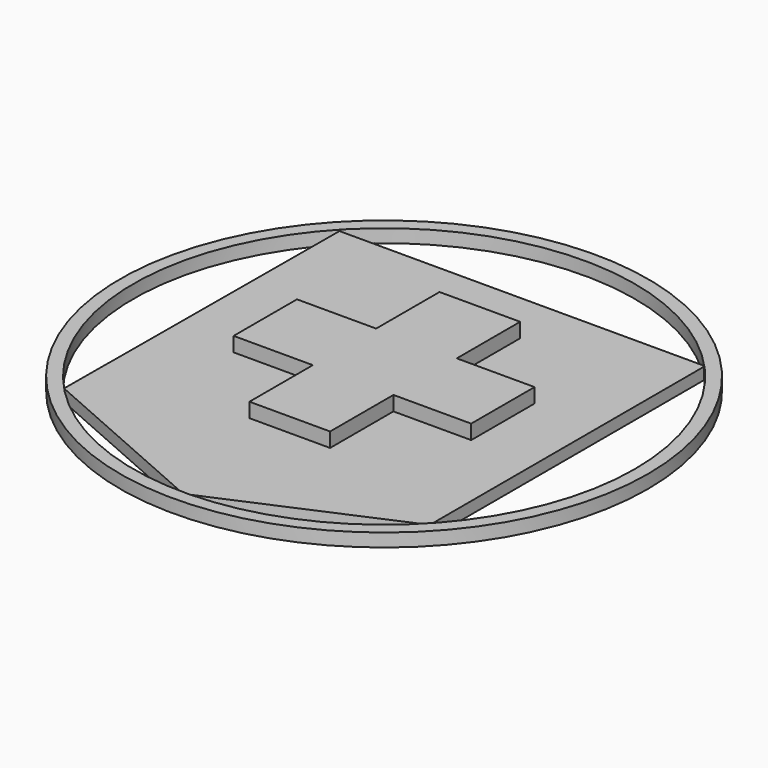
from build123d import *

# Parameters (mm, degrees)
F0_R     = 20
F0_R_2   = 19
F1_DEPTH = 1
F3_W     = 3
F3_H     = 3
F3_H_2   = 2.9973080382
F4_DEPTH = 2
F5_DEPTH = 0.9


with BuildPart() as f1:
    # F0 (on Top) → F1 (new body)
    with BuildSketch(Plane.XY):
        Circle(F0_R)
        Circle(F0_R_2, mode=Mode.SUBTRACT)
    extrude(amount=F1_DEPTH)


with BuildPart() as f4:
    # F3 (on Top) → F4 (new body)
    with BuildSketch(Plane.XY):
        Polygon((0, 2.9973080382), (0, 0), (3, 0), (3.1091126148, 0), (3.1091126148, 3), (0, 3), align=None)
        with Locations((-1.5, -1.5)):
            Rectangle(F3_W, F3_H)
        with Locations((-1.5, 1.4986540191)):
            Rectangle(F3_W, F3_H_2)
        Polygon((3, 0), (0, 0), (0, -3), (3.1091126148, -3), (3.1091126148, 0), align=None)
        Polygon((-3, -3), (-3, 0), (-3, 2.9973080382), (-9, 2.9973080382), (-9, -3), align=None)
        Polygon((-3, 2.9973080382), (0, 2.9973080382), (0, 3), (3.1091126148, 3), (3.1091126148, 9), (-3, 9), align=None)
        Polygon((3.1091126148, -3), (0, -3), (-3, -3), (-3, -9), (3.1091126148, -9), align=None)
        Polygon((3.1091126148, 3), (3.1091126148, 0), (3.1091126148, -3), (9, -3), (9, 3), align=None)
    extrude(amount=F4_DEPTH)

    # F2 (on Top) → F5 (join)
    with BuildSketch(Plane.XY):
        Polygon((13.8742914423, 13.047458604), (-13.8160753995, 13.047458604), (-13.9490468428, -12.8750633448), (0, -19.018009305), (13.8742914423, -13.0112969406), align=None)
    extrude(amount=F5_DEPTH)


solid = Compound([f1.part, f4.part])
